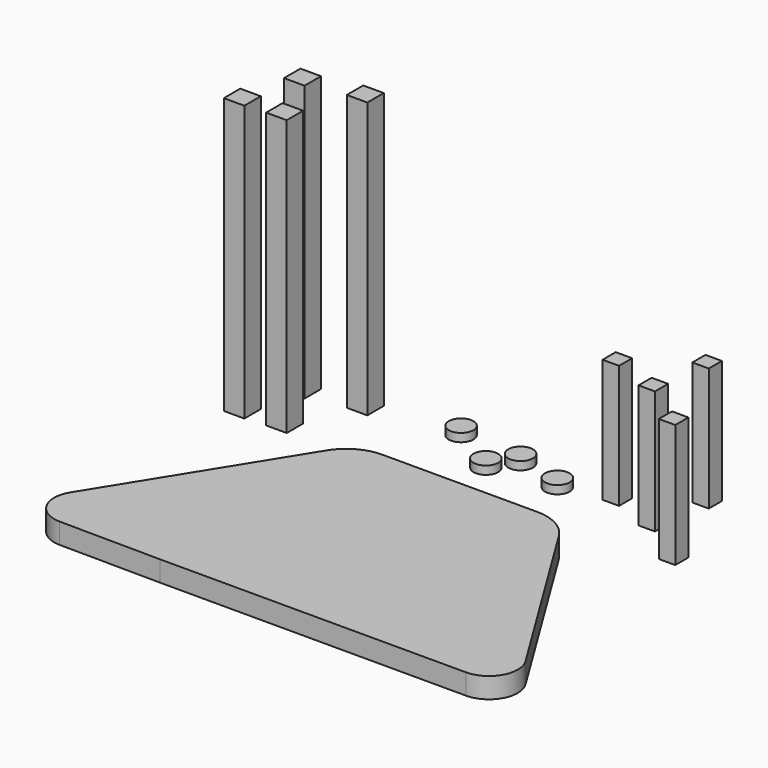
from build123d import *

# Parameters (mm, degrees)
F1_DEPTH = 6.35
F2_W     = 6.35
F2_H     = 6.35
F3_DEPTH = 85.09
F4_W     = 5.08
F4_H     = 5.08
F5_DEPTH = 38.1
F6_R     = 3.81
F8_DEPTH = 2.54


# Not quite as in the source:
# - the program builds the solid bodies; features that only make, move or delete a surface that nothing else refers to are left out


with BuildPart() as f1:
    # F0 (on Top) → F1 (new body)
    with BuildSketch(Plane.XY):
        with BuildLine():
            ThreePointArc((31.75, 35.721134447), (28.0284665024, 37.492055385), (23.9521475884, 38.1))
            Line((23.9521475884, 38.1), (-23.9740013608, 38.1))
            ThreePointArc((-23.9740013608, 38.1), (-28.0377301168, 37.4958897421), (-31.75, 35.7358065279))
            Line((-31.75, 35.7358065279), (-31.75, -38.1))
            Line((-31.75, -38.1), (31.75, -38.1))
            Line((31.75, -38.1), (31.75, 35.721134447))
        make_face()
        with BuildLine():
            Line((-31.75, -38.1), (-31.75, 35.7358065279))
            ThreePointArc((-31.75, 35.7358065279), (-34.0252899215, 33.8321903852), (-35.8473212157, 31.4910580505))
            Line((-35.8473212157, 31.4910580505), (-70.4080074235, -24.2550152634))
            ThreePointArc((-70.4080074235, -24.2550152634), (-70.6387165875, -33.2292164554), (-62.9295269359, -37.8289891312))
            Line((-62.9295269359, -37.8289891312), (-31.75, -38.1))
        make_face()
        with BuildLine():
            ThreePointArc((35.8430046385, 31.4626951809), (34.0241333068, 33.8107026443), (31.75, 35.721134447))
            Line((31.75, 35.721134447), (31.75, -38.1))
            Line((31.75, -38.1), (62.8297282478, -38.1))
            ThreePointArc((62.8297282478, -38.1), (70.5843439151, -33.5476304603), (70.3888780957, -24.5576401551))
            Line((70.3888780957, -24.5576401551), (35.8430046385, 31.4626951809))
        make_face()
    extrude(amount=F1_DEPTH)


with BuildPart() as f3:
    # F2 (on Top) → F3 (new body)
    with BuildSketch(Plane.XY):
        with Locations((-67.7386466112, 61.9670785964)):
            Rectangle(F2_W, F2_H)
    extrude(amount=F3_DEPTH)


with BuildPart() as f3b:
    # F2 (on Top) → F3, piece 2 (new body)
    with BuildSketch(Plane.XY):
        with Locations((-72.5461074233, 44.7328782558)):
            Rectangle(F2_W, F2_H)
    extrude(amount=F3_DEPTH)


with BuildPart() as f3c:
    # F2 (on Top) → F3, piece 3 (new body)
    with BuildSketch(Plane.XY):
        with Locations((-50.4183040082, 64.5559153438)):
            Rectangle(F2_W, F2_H)
    extrude(amount=F3_DEPTH)


with BuildPart() as f3d:
    # F2 (on Top) → F3, piece 4 (new body)
    with BuildSketch(Plane.XY):
        with Locations((-59.8461074233, 45.20164271)):
            Rectangle(F2_W, F2_H)
    extrude(amount=F3_DEPTH)


with BuildPart() as f5:
    # F4 (on Top) → F5 (new body)
    with BuildSketch(Plane.XY):
        with Locations((27.1672014992, 64.9249330163)):
            Rectangle(F4_W, F4_H)
    extrude(amount=F5_DEPTH)


with BuildPart() as f5b:
    # F4 (on Top) → F5, piece 2 (new body)
    with BuildSketch(Plane.XY):
        with Locations((44.959411025, 77.3479267955)):
            Rectangle(F4_W, F4_H)
    extrude(amount=F5_DEPTH)


with BuildPart() as f5c:
    # F4 (on Top) → F5, piece 3 (new body)
    with BuildSketch(Plane.XY):
        with Locations((42.2973409295, 59.8965808749)):
            Rectangle(F4_W, F4_H)
    extrude(amount=F5_DEPTH)


with BuildPart() as f5d:
    # F4 (on Top) → F5, piece 4 (new body)
    with BuildSketch(Plane.XY):
        with Locations((57.0866167545, 49.2483004928)):
            Rectangle(F4_W, F4_H)
    extrude(amount=F5_DEPTH)


with BuildPart() as f8:
    # F6 (on Top) → F8 (new body)
    with BuildSketch(Plane.XY):
        with Locations((-2.7939286083, 64.9956390262)):
            Circle(F6_R)
    extrude(amount=F8_DEPTH)


with BuildPart() as f8b:
    # F6 (on Top) → F8, piece 2 (new body)
    with BuildSketch(Plane.XY):
        with Locations((11.9659397751, 60.7509315014)):
            Circle(F6_R)
    extrude(amount=F8_DEPTH)


with BuildPart() as f8c:
    # F6 (on Top) → F8, piece 3 (new body)
    with BuildSketch(Plane.XY):
        with Locations((-7.8719547018, 57.932112366)):
            Circle(F6_R)
    extrude(amount=F8_DEPTH)


with BuildPart() as f8d:
    # F6 (on Top) → F8, piece 4 (new body)
    with BuildSketch(Plane.XY):
        with Locations((-23.1860335916, 67.5050541759)):
            Circle(F6_R)
    extrude(amount=F8_DEPTH)


solid = Compound([f1.part, f3.part, f3b.part, f3c.part, f3d.part, f5.part, f5b.part, f5c.part, f5d.part, f8.part, f8b.part, f8c.part, f8d.part])
